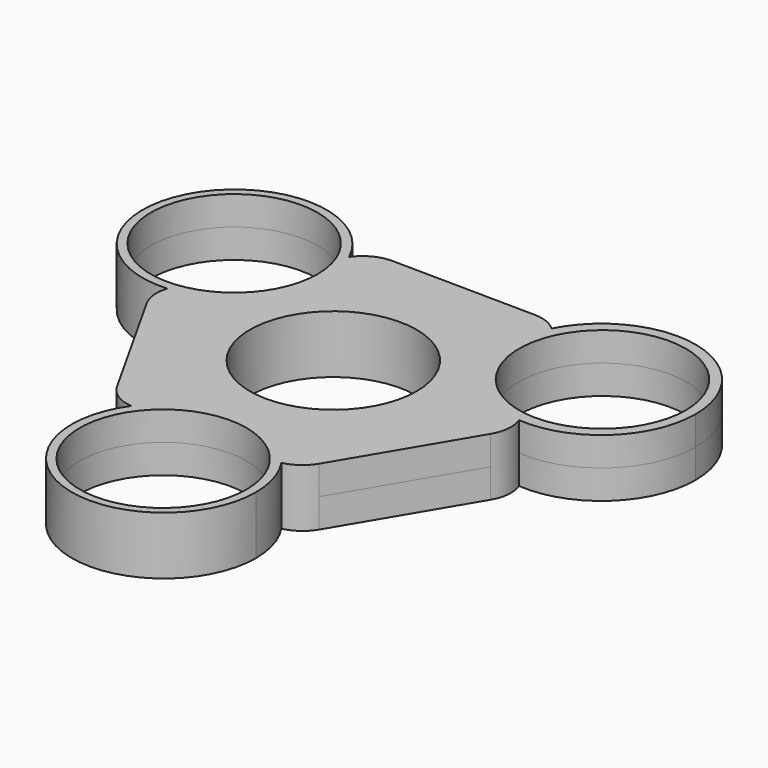
from build123d import *

# Parameters (mm, degrees)
F2_DEPTH     = 4
F0_R         = 11.5
F3_DEPTH     = 4
F4_T1_DEPTH  = 21.9483713996
F4_T3_DEPTH  = 22.3459559115
F4_T5_DEPTH  = 21.2495705846
F4_T7_DEPTH  = 22.5954800676
F4_T9_DEPTH  = 22.5954384353
F4_T11_DEPTH = 21.948545213


# Not quite as in the source:
# - a fillet or chamfer that OpenCascade refuses, or shapes differently, is made with other operations: its cross-section is extruded or revolved along the edge and cut away or added


with BuildPart() as f2:
    # F1 (on Top) → F2 (new body, symmetric)
    with BuildSketch(Plane.XY):
        with BuildLine():
            ThreePointArc((-24.434154737, 1.9297075548), (-16.0117202716, 5.9282775779), (-12.5894382026, 14.6008752276))
            ThreePointArc((-12.5894382026, 14.6008752276), (-12.8847624083, 17.3237447508), (-13.7570001617, 19.9199797418))
            Line((-13.7570001617, 19.9199797418), (-24.434154737, 1.9297075548))
        make_face()
        with BuildLine():
            ThreePointArc((-13.7570001617, 19.9199797418), (-12.8847624083, 17.3237447508), (-12.5894382026, 14.6008752276))
            ThreePointArc((-12.5894382026, 14.6008752276), (-16.0117202716, 5.9282775779), (-24.434154737, 1.9297075548))
            Line((-24.434154737, 1.9297075548), (-25.3981637022, 0.3054186533))
            Line((-25.3981637022, 0.3054186533), (-12.9635821636, -21.842745649))
            Line((-12.9635821636, -21.842745649), (-10.3728090059, -21.8739002812))
            ThreePointArc((-10.3728090059, -21.8739002812), (0.1527093266, -16.5024942777), (10.54601793, -22.1254538984))
            Line((10.54601793, -22.1254538984), (12.4345815386, -22.1481643023))
            Line((12.4345815386, -22.1481643023), (25.3981637022, -0.3054186533))
            Line((25.3981637022, -0.3054186533), (24.3123835544, 1.6285456733))
            ThreePointArc((24.3123835544, 1.6285456733), (13.9458157922, 8.2323089444), (13.7055148895, 20.5212337137))
            Line((13.7055148895, 20.5212337137), (12.9635821636, 21.842745649))
            Line((12.9635821636, 21.842745649), (-12.4345815386, 22.1481643023))
            Line((-12.4345815386, 22.1481643023), (-13.7570001617, 19.9199797418))
        make_face()
        with BuildLine():
            Line((-24.434154737, 1.9297075548), (-13.7570001617, 19.9199797418))
            ThreePointArc((-13.7570001617, 19.9199797418), (-36.2108110271, 21.0826663094), (-24.434154737, 1.9297075548))
        make_face()
        with BuildLine():
            Line((24.3123835544, 1.6285456733), (13.7055148895, 20.5212337137))
            ThreePointArc((13.7055148895, 20.5212337137), (13.9458157922, 8.2323089444), (24.3123835544, 1.6285456733))
        make_face()
        with BuildLine():
            ThreePointArc((38.29859269, 14.6009373546), (28.3341688507, 27.2487571734), (13.7055148895, 20.5212337137))
            Line((13.7055148895, 20.5212337137), (24.3123835544, 1.6285456733))
            ThreePointArc((24.3123835544, 1.6285456733), (34.136115438, 5.0628952085), (38.29859269, 14.6009373546))
        make_face()
        with BuildLine():
            Line((10.54601793, -22.1254538984), (-10.3728090059, -21.8739002812))
            ThreePointArc((-10.3728090059, -21.8739002812), (-3.8441725784, -41.3058041995), (12.7, -29.2015761288))
            ThreePointArc((12.7, -29.2015761288), (12.1495766945, -25.5032270182), (10.54601793, -22.1254538984))
        make_face()
        with BuildLine():
            ThreePointArc((10.54601793, -22.1254538984), (0.1527093266, -16.5024942777), (-10.3728090059, -21.8739002812))
            Line((-10.3728090059, -21.8739002812), (10.54601793, -22.1254538984))
        make_face()
    extrude(amount=F2_DEPTH, both=True)

    # F0 (on Top) → F3 (cut, symmetric)
    with BuildSketch(Plane.XY):
        with Locations((-25.4, 14.6646968374)):
            Circle(F0_R)
        with Locations((25.4, 14.6646968374)):
            Circle(F0_R)
        with Locations((0, -29.3293936748)):
            Circle(F0_R)
        Circle(F0_R)
    extrude(amount=F3_DEPTH, both=True, mode=Mode.SUBTRACT)

    # F4: fillet of radius 5.08 on 6 edges, made by hand

    # F4_s2 → F4_t1 (cut)
    with BuildSketch(Plane.XY.offset(-10.9741856998)):
        with BuildLine():
            ThreePointArc((10.54601793, -22.1254538984), (12.4510077343, -21.2841478503), (13.8583678275, -19.7491821865))
            Line((13.8583678275, -19.7491821865), (12.4345815386, -22.1481643023))
            Line((12.4345815386, -22.1481643023), (10.54601793, -22.1254538984))
        make_face()
    extrude(amount=F4_T1_DEPTH, mode=Mode.SUBTRACT)

    # F4_s4 → F4_t3 (cut)
    with BuildSketch(Plane.XY.offset(-11.1729779558)):
        with BuildLine():
            ThreePointArc((23.9337937954, -2.7727813782), (24.6265549669, -0.6154246052), (24.3123835544, 1.6285456733))
            Line((24.3123835544, 1.6285456733), (25.3981637022, -0.3054186533))
            Line((25.3981637022, -0.3054186533), (23.9337937954, -2.7727813782))
        make_face()
    extrude(amount=F4_T3_DEPTH, mode=Mode.SUBTRACT)

    # F4_s6 → F4_t5 (cut)
    with BuildSketch(Plane.XY.offset(-10.6247852923)):
        with BuildLine():
            ThreePointArc((10.3138596228, 21.8746091608), (12.1354983401, 21.5132129748), (13.7055148895, 20.5212337137))
            Line((13.7055148895, 20.5212337137), (12.9635821636, 21.842745649))
            Line((12.9635821636, 21.842745649), (10.3138596228, 21.8746091608))
        make_face()
    extrude(amount=F4_T5_DEPTH, mode=Mode.SUBTRACT)

    # F4_s8 → F4_t7 (cut)
    with BuildSketch(Plane.XY.offset(-11.2977400338)):
        with BuildLine():
            ThreePointArc((-13.7570001617, 19.9199797418), (-11.910066672, 21.54587795), (-9.5156965617, 22.1130640513))
            Line((-9.5156965617, 22.1130640513), (-12.4345815386, 22.1481643023))
            Line((-12.4345815386, 22.1481643023), (-13.7570001617, 19.9199797418))
        make_face()
    extrude(amount=F4_T7_DEPTH, mode=Mode.SUBTRACT)

    # F4_s10 → F4_t9 (cut)
    with BuildSketch(Plane.XY.offset(-11.2977192176)):
        with BuildLine():
            ThreePointArc((-14.3926228669, -19.2973742433), (-12.7042844419, -21.0873382025), (-10.3728090059, -21.8739002812))
            Line((-10.3728090059, -21.8739002812), (-12.9635821636, -21.842745649))
            Line((-12.9635821636, -21.842745649), (-14.3926228669, -19.2973742433))
        make_face()
    extrude(amount=F4_T9_DEPTH, mode=Mode.SUBTRACT)

    # F4_s12 → F4_t11 (cut)
    with BuildSketch(Plane.XY.offset(-10.9742726065)):
        with BuildLine():
            ThreePointArc((-24.0324603731, -2.1271378125), (-24.6581063385, -0.1407771898), (-24.434154737, 1.9297075548))
            Line((-24.434154737, 1.9297075548), (-25.3981637022, 0.3054186533))
            Line((-25.3981637022, 0.3054186533), (-24.0324603731, -2.1271378125))
        make_face()
    extrude(amount=F4_T11_DEPTH, mode=Mode.SUBTRACT)


solid = f2.part
